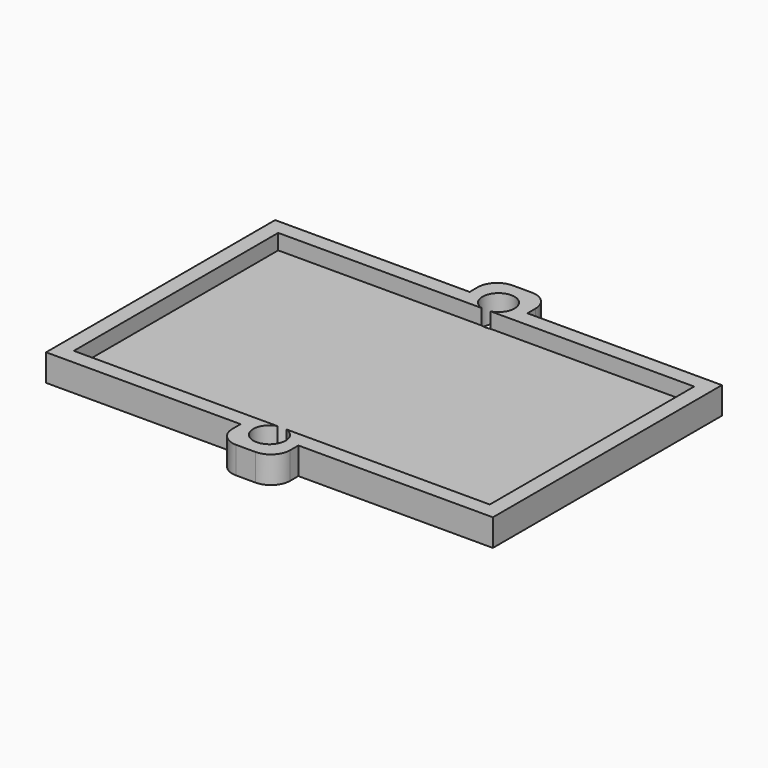
from build123d import *

# Parameters (mm, degrees)
F1_DEPTH = 2.4
F0_W     = 60
F0_H     = 35
F2_DEPTH = 1.8


# Not quite as in the source:
# - ends of sketch curves that miss each other by under 0.0002 mm in the source are joined


with BuildPart() as f1:
    # F0 (on Top) → F1 (new body)
    with BuildSketch(Plane.XY):
        Polygon((-32.7, -16.904), (-32.7, 22.896), (-4.8, 22.896), (-4.8, 25.2960002601), (-35.1000002601, 25.2960002601), (-35.1000002601, -19.3040002601), (-4.8, -19.3040002601), (-4.8, -16.904), align=None)
        Polygon((4.2, 25.2960002601), (4.2, 22.896), (32.1, 22.896), (32.1, -16.904), (4.2, -16.904), (4.2, -19.3040002601), (34.5000002601, -19.3040002601), (34.5000002601, 25.2960002601), align=None)
        with BuildLine():
            ThreePointArc((2.2, 25.296), (1.7, 23.796), (0.4, 22.896))
            Line((0.4, 22.896), (4.2, 22.896))
            Line((4.2, 22.896), (4.2, 25.2960002601))
            Line((4.2, 25.2960002601), (2.2, 25.296))
        make_face()
        with BuildLine():
            Line((-4.8, 25.2960002601), (-4.8, 22.896))
            Line((-4.8, 22.896), (-1, 22.896))
            ThreePointArc((-1, 22.896), (-2.300000078, 23.796000104), (-2.8, 25.2960002601))
            Line((-2.8, 25.2960002601), (-4.8, 25.2960002601))
        make_face()
        with BuildLine():
            Line((-4.8, 26.896), (-4.8, 25.2960002601))
            Line((-4.8, 25.2960002601), (-2.8, 25.2960002601))
            ThreePointArc((-2.8, 25.2960002601), (-0.2999998699, 27.796), (2.2, 25.296))
            Line((2.2, 25.296), (4.2, 25.2960002601))
            Line((4.2, 25.2960002601), (4.2, 26.896))
            ThreePointArc((4.2, 26.896), (3.3213203436, 29.0173203436), (1.2, 29.896))
            Line((1.2, 29.896), (-1.8, 29.896))
            ThreePointArc((-1.8, 29.896), (-3.9213203436, 29.0173203436), (-4.8, 26.896))
        make_face()
        with BuildLine():
            Line((-1, -16.904), (-4.8, -16.904))
            Line((-4.8, -16.904), (-4.8, -19.3040002601))
            Line((-4.8, -19.3040002601), (-4.8, -20.904))
            ThreePointArc((-4.8, -20.904), (-3.9213203436, -23.0253203436), (-1.8, -23.904))
            Line((-1.8, -23.904), (1.2, -23.904))
            ThreePointArc((1.2, -23.904), (3.3213203436, -23.0253203436), (4.2, -20.904))
            Line((4.2, -20.904), (4.2, -19.3040002601))
            Line((4.2, -19.3040002601), (4.2, -16.904))
            Line((4.2, -16.904), (0.4, -16.904))
            ThreePointArc((0.4, -16.904), (1.7, -17.804), (2.2, -19.304))
            ThreePointArc((2.2, -19.304), (-1.8, -21.304), (-1, -16.904))
        make_face()
    extrude(amount=F1_DEPTH)

    # F0 (on Top) → F2 (join)
    with BuildSketch(Plane.XY):
        Polygon((4.2, 25.2960002601), (4.2, 22.896), (32.1, 22.896), (32.1, -16.904), (4.2, -16.904), (4.2, -19.3040002601), (34.5000002601, -19.3040002601), (34.5000002601, 25.2960002601), align=None)
        with BuildLine():
            Line((-4.8, 22.896), (-32.7, 22.896))
            Line((-32.7, 22.896), (-32.7, -16.904))
            Line((-32.7, -16.904), (-4.8, -16.904))
            Line((-4.8, -16.904), (-1, -16.904))
            ThreePointArc((-1, -16.904), (-0.3, -16.804), (0.4, -16.904))
            Line((0.4, -16.904), (4.2, -16.904))
            Line((4.2, -16.904), (32.1, -16.904))
            Line((32.1, -16.904), (32.1, 22.896))
            Line((32.1, 22.896), (4.2, 22.896))
            Line((4.2, 22.896), (0.4, 22.896))
            ThreePointArc((0.4, 22.896), (-0.3, 22.796), (-1, 22.896))
            Line((-1, 22.896), (-4.8, 22.896))
        make_face()
        with Locations((-0.3, 2.996)):
            Rectangle(F0_W, F0_H, mode=Mode.SUBTRACT)
        with Locations((-0.3, 2.996)):
            Rectangle(F0_W, F0_H)
        Polygon((-32.7, -16.904), (-32.7, 22.896), (-4.8, 22.896), (-4.8, 25.2960002601), (-35.1000002601, 25.2960002601), (-35.1000002601, -19.3040002601), (-4.8, -19.3040002601), (-4.8, -16.904), align=None)
        with BuildLine():
            Line((-1, -16.904), (-4.8, -16.904))
            Line((-4.8, -16.904), (-4.8, -19.3040002601))
            Line((-4.8, -19.3040002601), (-4.8, -20.904))
            ThreePointArc((-4.8, -20.904), (-3.9213203436, -23.0253203436), (-1.8, -23.904))
            Line((-1.8, -23.904), (1.2, -23.904))
            ThreePointArc((1.2, -23.904), (3.3213203436, -23.0253203436), (4.2, -20.904))
            Line((4.2, -20.904), (4.2, -19.3040002601))
            Line((4.2, -19.3040002601), (4.2, -16.904))
            Line((4.2, -16.904), (0.4, -16.904))
            ThreePointArc((0.4, -16.904), (1.7, -17.804), (2.2, -19.304))
            ThreePointArc((2.2, -19.304), (-1.8, -21.304), (-1, -16.904))
        make_face()
        with BuildLine():
            Line((-4.8, 26.896), (-4.8, 25.2960002601))
            Line((-4.8, 25.2960002601), (-2.8, 25.2960002601))
            ThreePointArc((-2.8, 25.2960002601), (-0.2999998699, 27.796), (2.2, 25.296))
            Line((2.2, 25.296), (4.2, 25.2960002601))
            Line((4.2, 25.2960002601), (4.2, 26.896))
            ThreePointArc((4.2, 26.896), (3.3213203436, 29.0173203436), (1.2, 29.896))
            Line((1.2, 29.896), (-1.8, 29.896))
            ThreePointArc((-1.8, 29.896), (-3.9213203436, 29.0173203436), (-4.8, 26.896))
        make_face()
        with BuildLine():
            ThreePointArc((2.2, 25.296), (1.7, 23.796), (0.4, 22.896))
            Line((0.4, 22.896), (4.2, 22.896))
            Line((4.2, 22.896), (4.2, 25.2960002601))
            Line((4.2, 25.2960002601), (2.2, 25.296))
        make_face()
        with BuildLine():
            Line((-4.8, 25.2960002601), (-4.8, 22.896))
            Line((-4.8, 22.896), (-1, 22.896))
            ThreePointArc((-1, 22.896), (-2.300000078, 23.796000104), (-2.8, 25.2960002601))
            Line((-2.8, 25.2960002601), (-4.8, 25.2960002601))
        make_face()
    extrude(amount=-F2_DEPTH)


solid = f1.part
